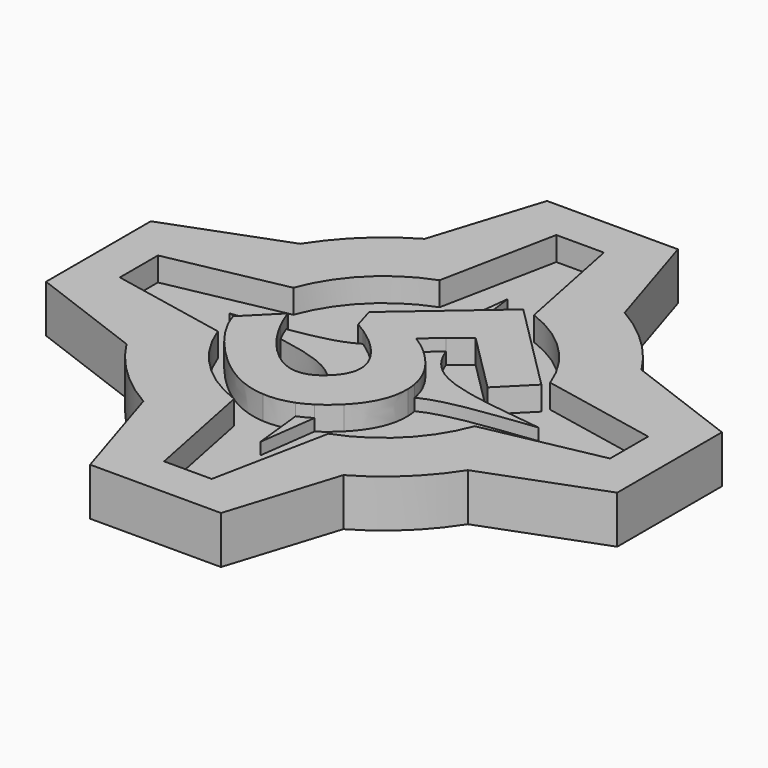
from build123d import *

# Parameters (mm, degrees)
F1_DEPTH = 2
F2_DEPTH = 1
F3_DEPTH = 1.5


# Not quite as in the source:
# - a feature names something its author has since deleted; it is built from what else it names


with BuildPart() as f1:
    # F0 (on Top) → F1 (new body)
    with BuildSketch(Plane.XY):
        with BuildLine():
            Line((-2.75, 12), (-4.2021191449, 7.3886531041))
            ThreePointArc((-4.2021191449, 7.3886531041), (-5.8600472341, 6.1570972393), (-7.1720131073, 4.5620420853))
            Line((-7.1720131073, 4.5620420853), (-12, 2.75))
            Line((-12, 2.75), (-12, -2.75))
            Line((-12, -2.75), (-7.1720131073, -4.5620420853))
            ThreePointArc((-7.1720131073, -4.5620420853), (-5.8600472341, -6.1570972393), (-4.2021191449, -7.3886531041))
            Line((-4.2021191449, -7.3886531041), (-2.75, -12))
            Line((-2.75, -12), (2.75, -12))
            Line((2.75, -12), (4.2021191449, -7.3886531041))
            ThreePointArc((4.2021191449, -7.3886531041), (5.8600472341, -6.1570972393), (7.1720131073, -4.5620420853))
            Line((7.1720131073, -4.5620420853), (12, -2.75))
            Line((12, -2.75), (12, 2.75))
            Line((12, 2.75), (7.1720131073, 4.5620420853))
            ThreePointArc((7.1720131073, 4.5620420853), (5.8600472341, 6.1570972393), (4.2021191449, 7.3886531041))
            Line((4.2021191449, 7.3886531041), (2.75, 12))
            Line((2.75, 12), (-2.75, 12))
        make_face()
        with BuildLine():
            ThreePointArc((-5.3974610581, 1.9824011012), (-4.0658639918, 4.0658639918), (-1.9824011012, 5.3974610581))
            Line((-1.9824011012, 5.3974610581), (-1, 10.3))
            Line((-1, 10.3), (1, 10.3))
            Line((1, 10.3), (1.9824011012, 5.3974610581))
            ThreePointArc((1.9824011012, 5.3974610581), (4.0658639918, 4.0658639918), (5.3974610581, 1.9824011012))
            Line((5.3974610581, 1.9824011012), (10.3, 1))
            Line((10.3, 1), (10.3, -1))
            Line((10.3, -1), (5.3974610581, -1.9824011012))
            ThreePointArc((5.3974610581, -1.9824011012), (4.0658639918, -4.0658639918), (1.9824011012, -5.3974610581))
            Line((1.9824011012, -5.3974610581), (1, -10.3))
            Line((1, -10.3), (-1, -10.3))
            Line((-1, -10.3), (-1.9824011012, -5.3974610581))
            ThreePointArc((-1.9824011012, -5.3974610581), (-4.0658639918, -4.0658639918), (-5.3974610581, -1.9824011012))
            Line((-5.3974610581, -1.9824011012), (-10.3, -1))
            Line((-10.3, -1), (-10.3, 1))
            Line((-10.3, 1), (-5.3974610581, 1.9824011012))
        make_face(mode=Mode.SUBTRACT)
    extrude(amount=F1_DEPTH)


with BuildPart() as f1b:
    # F0 (on Top) → F1, piece 2 (new body)
    with BuildSketch(Plane.XY):
        with BuildLine():
            Line((1.4579168065, 5.4941121132), (0.2654571044, 4.46607152))
            add(Edge.make_bspline(
                [(0.7478959675, 2.3141081763), (0.5408536455, 2.8552696341), (0.3998514188, 3.5527800211), (0.2654571044, 4.46607152)],
                knots=[6.0401561985, 6.0401561985, 6.0401561985, 6.0401561985, 7.9623527609, 7.9623527609, 7.9623527609, 7.9623527609], degree=3))
            Line((0.7478959675, 2.3141081763), (1.5004693947, 2.9375949951))
            Line((1.5004693947, 2.9375949951), (4.0028660863, 0.4343877588))
            Line((4.0028660863, 0.4343877588), (5.2598413938, 1.6909560547))
            Line((5.2598413938, 1.6909560547), (1.4579168065, 5.4941121132))
        make_face()
        with BuildLine():
            add(Edge.make_bspline(
                [(-0.7099336682, -2.2396454304), (-0.6256818584, -2.1704916087), (-0.5427903728, -2.0876269636)],
                knots=[0.925504666, 0.925504666, 0.925504666, 1, 1, 1], degree=2))
            add(Edge.make_bspline(
                [(-0.7099336682, -2.2396454304), (-0.4881454517, -2.7630250257), (-0.3518820462, -3.4434694111), (-0.2338863041, -4.3482357339)],
                knots=[5.8413396547, 5.8413396547, 5.8413396547, 5.8413396547, 7.8444431249, 7.8444431249, 7.8444431249, 7.8444431249], degree=3))
            add(Edge.make_bspline(
                [(0.3290608575, -4.0601655454), (0.0522382207, -4.2361734258), (-0.2338863041, -4.3482357339)],
                knots=[0.309252581, 0.309252581, 0.309252581, 0.5341322792, 0.5341322792, 0.5341322792], degree=2))
            add(Edge.make_bspline(
                [(0.3290608575, -4.0601655454), (0.6228480721, -2.2554562931), (0.987071243, -1.3852263771), (1.9925938258, -0.8786123417)],
                knots=[1.5244578408, 1.5244578408, 1.5244578408, 1.5244578408, 5.6104856332, 5.6104856332, 5.6104856332, 5.6104856332], degree=3))
            add(Edge.make_bspline(
                [(0.987609764, 0.8998355547), (1.8233684173, 0.0638061932), (1.9925938258, -0.8786123417)],
                knots=[0, 0, 0, 0.8228500432, 0.8228500432, 0.8228500432], degree=2))
            add(Edge.make_bspline(
                [(0.1959038432, 1.5567382899), (0.556479494, 1.331105471), (0.987609764, 0.8998355547)],
                knots=[0, 0, 0, 1, 1, 1], degree=2))
            Line((0.1959038432, 1.5567382899), (-0.0050966464, 1.6902740726))
            Line((-0.0050966464, 1.6902740726), (0.7478959675, 2.3141081763))
            add(Edge.make_bspline(
                [(0.7478959675, 2.3141081763), (0.5408536455, 2.8552696341), (0.3998514188, 3.5527800211), (0.2654571044, 4.46607152)],
                knots=[6.0401561985, 6.0401561985, 6.0401561985, 6.0401561985, 7.9623527609, 7.9623527609, 7.9623527609, 7.9623527609], degree=3))
            Line((0.2654571044, 4.46607152), (-0.3272992398, 3.9550457951))
            add(Edge.make_bspline(
                [(-0.3272992398, 3.9550457951), (-0.5803192593, 2.3906018232), (-0.9091205356, 1.5574827335), (-1.7244009065, 1.0449906882)],
                knots=[1.621694993, 1.621694993, 1.621694993, 1.621694993, 5.2829617669, 5.2829617669, 5.2829617669, 5.2829617669], degree=3))
            add(Edge.make_bspline(
                [(-1.4983144688, 0.8879619345), (-1.6173066461, 0.9732773429), (-1.7244009065, 1.0449906882)],
                knots=[0, 0, 0, 0.3328437229, 0.3328437229, 0.3328437229], degree=2))
            add(Edge.make_bspline(
                [(-0.8876580426, 0.3784024309), (-1.1408128274, 0.6316392144), (-1.4983144688, 0.8879619345)],
                knots=[0, 0, 0, 1, 1, 1], degree=2))
            add(Edge.make_bspline(
                [(-0.5427903728, -2.0876269636), (0.5177345813, -1.02744541), (-0.8876580426, 0.3784024309)],
                knots=[0, 0, 0, 1, 1, 1], degree=2))
        make_face()
        with BuildLine():
            add(Edge.make_bspline(
                [(-1.7244009065, 1.0449906882), (-1.9390620317, 1.1887338482), (-2.1059212368, 1.2778283886)],
                knots=[0.3328437229, 0.3328437229, 0.3328437229, 1, 1, 1], degree=2))
            add(Edge.make_bspline(
                [(-0.3272992398, 3.9550457951), (-0.5803192593, 2.3906018232), (-0.9091205356, 1.5574827335), (-1.7244009065, 1.0449906882)],
                knots=[1.621694993, 1.621694993, 1.621694993, 1.621694993, 5.2829617669, 5.2829617669, 5.2829617669, 5.2829617669], degree=3))
            Line((-0.3272992398, 3.9550457951), (-2.3789186791, 2.1863084016))
            Line((-2.3789186791, 2.1863084016), (-2.1059212368, 1.2778283886))
        make_face()
        with BuildLine():
            add(Edge.make_bspline(
                [(0.3290608575, -4.0601655454), (0.6228480721, -2.2554562931), (0.987071243, -1.3852263771), (1.9925938258, -0.8786123417)],
                knots=[1.5244578408, 1.5244578408, 1.5244578408, 1.5244578408, 5.6104856332, 5.6104856332, 5.6104856332, 5.6104856332], degree=3))
            add(Edge.make_bspline(
                [(1.07283769, -3.4551458487), (0.7097449104, -3.818121058), (0.3290608575, -4.0601655454)],
                knots=[0, 0, 0, 0.309252581, 0.309252581, 0.309252581], degree=2))
            add(Edge.make_bspline(
                [(2.0345651408, -1.289326677), (2.0658328352, -2.4624722377), (1.07283769, -3.4551458487)],
                knots=[0, 0, 0, 1, 1, 1], degree=2))
            add(Edge.make_bspline(
                [(1.9925938258, -0.8786123417), (2.0290260701, -1.0815039915), (2.0345651408, -1.289326677)],
                knots=[0.8228500432, 0.8228500432, 0.8228500432, 1, 1, 1], degree=2))
        make_face()
        with BuildLine():
            add(Edge.make_bspline(
                [(-5.0476920503, -0.2054319436), (-4.6911689085, -0.2581182841), (-4.3627018531, -0.3095354756), (-4.0598230569, -0.3621513456)],
                knots=[0.8212011644, 0.8212011644, 0.8212011644, 0.8212011644, 1.4868249386, 1.4868249386, 1.4868249386, 1.4868249386], degree=3))
            Line((-5.0476920503, -0.2054319436), (-5.6740216756, -0.8315587618))
            add(Edge.make_bspline(
                [(-4.1644213444, -3.0998236856), (-5.3350704405, -1.9287954077), (-5.6740216756, -0.8315587618)],
                knots=[0, 0, 0, 1, 1, 1], degree=2))
            add(Edge.make_bspline(
                [(-1.4592955796, -4.5381069077), (-2.8173310346, -4.4473503278), (-4.1644213444, -3.0998236856)],
                knots=[0, 0, 0, 1, 1, 1], degree=2))
            add(Edge.make_bspline(
                [(-0.2338863041, -4.3482357339), (-0.8266306975, -4.5803874688), (-1.4592955796, -4.5381069077)],
                knots=[0.5341322792, 0.5341322792, 0.5341322792, 1, 1, 1], degree=2))
            add(Edge.make_bspline(
                [(-0.7099336682, -2.2396454304), (-0.4881454517, -2.7630250257), (-0.3518820462, -3.4434694111), (-0.2338863041, -4.3482357339)],
                knots=[5.8413396547, 5.8413396547, 5.8413396547, 5.8413396547, 7.8444431249, 7.8444431249, 7.8444431249, 7.8444431249], degree=3))
            add(Edge.make_bspline(
                [(-3.0133276619, -1.8417037247), (-1.7566494671, -3.0987889667), (-0.7099336682, -2.2396454304)],
                knots=[0, 0, 0, 0.925504666, 0.925504666, 0.925504666], degree=2))
            add(Edge.make_bspline(
                [(-3.8394915756, -0.7605006452), (-3.4628691889, -1.3920165878), (-3.0133276619, -1.8417037247)],
                knots=[0, 0, 0, 1, 1, 1], degree=2))
            add(Edge.make_bspline(
                [(-4.0598230569, -0.3621513456), (-3.9598892689, -0.5586192237), (-3.8394915756, -0.7605006452)],
                knots=[0.6803225258, 0.6803225258, 0.6803225258, 1, 1, 1], degree=2))
        make_face()
        with BuildLine():
            Line((-4.5875235257, 0.2545875773), (-5.0476920503, -0.2054319436))
            add(Edge.make_bspline(
                [(-5.0476920503, -0.2054319436), (-4.6911689085, -0.2581182841), (-4.3627018531, -0.3095354756), (-4.0598230569, -0.3621513456)],
                knots=[0.8212011644, 0.8212011644, 0.8212011644, 0.8212011644, 1.4868249386, 1.4868249386, 1.4868249386, 1.4868249386], degree=3))
            add(Edge.make_bspline(
                [(-4.3409756358, 0.2916852868), (-4.2301083517, -0.0273737774), (-4.0598230569, -0.3621513456)],
                knots=[0.1355981238, 0.1355981238, 0.1355981238, 0.6803225258, 0.6803225258, 0.6803225258], degree=2))
            add(Edge.make_bspline(
                [(-4.3409756358, 0.2916852868), (-4.4214269269, 0.2792690242), (-4.5035953579, 0.26691732), (-4.5875235257, 0.2545875773)],
                knots=[7.8805599952, 7.8805599952, 7.8805599952, 7.8805599952, 8.0525816561, 8.0525816561, 8.0525816561, 8.0525816561], degree=3))
        make_face()
        with BuildLine():
            Line((-4.3924900739, 0.4495578768), (-4.5875235257, 0.2545875773))
            add(Edge.make_bspline(
                [(-4.3409756358, 0.2916852868), (-4.4214269269, 0.2792690242), (-4.5035953579, 0.26691732), (-4.5875235257, 0.2545875773)],
                knots=[7.8805599952, 7.8805599952, 7.8805599952, 7.8805599952, 8.0525816561, 8.0525816561, 8.0525816561, 8.0525816561], degree=3))
            add(Edge.make_bspline(
                [(-4.3924900739, 0.4495578768), (-4.3685738041, 0.3711085885), (-4.3409756358, 0.2916852868)],
                knots=[0, 0, 0, 0.1355981238, 0.1355981238, 0.1355981238], degree=2))
        make_face()
    extrude(amount=F1_DEPTH)


with BuildPart() as f2:
    # F0 (on Top) → F2 (new body)
    with BuildSketch(Plane.XY):
        with BuildLine():
            Line((-1, 10.3), (-1.9824011012, 5.3974610581))
            ThreePointArc((-1.9824011012, 5.3974610581), (-4.0658639918, 4.0658639918), (-5.3974610581, 1.9824011012))
            Line((-5.3974610581, 1.9824011012), (-10.3, 1))
            Line((-10.3, 1), (-10.3, -1))
            Line((-10.3, -1), (-5.3974610581, -1.9824011012))
            ThreePointArc((-5.3974610581, -1.9824011012), (-4.0658639918, -4.0658639918), (-1.9824011012, -5.3974610581))
            Line((-1.9824011012, -5.3974610581), (-1, -10.3))
            Line((-1, -10.3), (1, -10.3))
            Line((1, -10.3), (1.9824011012, -5.3974610581))
            ThreePointArc((1.9824011012, -5.3974610581), (4.0658639918, -4.0658639918), (5.3974610581, -1.9824011012))
            Line((5.3974610581, -1.9824011012), (10.3, -1))
            Line((10.3, -1), (10.3, 1))
            Line((10.3, 1), (5.3974610581, 1.9824011012))
            ThreePointArc((5.3974610581, 1.9824011012), (4.0658639918, 4.0658639918), (1.9824011012, 5.3974610581))
            Line((1.9824011012, 5.3974610581), (1, 10.3))
            Line((1, 10.3), (-1, 10.3))
        make_face()
        with BuildLine():
            add(Edge.make_bspline(
                [(-6.5, 0), (-5.9701038682, -0.0734985607), (-5.4875459594, -0.1404311341), (-5.0476920503, -0.2054319436)],
                knots=[0, 0, 0, 0, 0.8212011644, 0.8212011644, 0.8212011644, 0.8212011644], degree=3))
            add(Edge.make_bspline(
                [(-4.5875235257, 0.2545875773), (-5.1436271619, 0.1728913493), (-5.7769888409, 0.0921593026), (-6.5, 0)],
                knots=[8.0525816561, 8.0525816561, 8.0525816561, 8.0525816561, 9.1923881554, 9.1923881554, 9.1923881554, 9.1923881554], degree=3))
            Line((-4.5875235257, 0.2545875773), (-4.3924900739, 0.4495578768))
            add(Edge.make_bspline(
                [(-4.3924900739, 0.4495578768), (-4.3685738041, 0.3711085885), (-4.3409756358, 0.2916852868)],
                knots=[0, 0, 0, 0.1355981238, 0.1355981238, 0.1355981238], degree=2))
            add(Edge.make_bspline(
                [(-1.7244009065, 1.0449906882), (-2.3028266202, 0.6813874572), (-3.1261278658, 0.4791759876), (-4.3409756358, 0.2916852868)],
                knots=[5.2829617669, 5.2829617669, 5.2829617669, 5.2829617669, 7.8805599952, 7.8805599952, 7.8805599952, 7.8805599952], degree=3))
            add(Edge.make_bspline(
                [(-1.7244009065, 1.0449906882), (-1.9390620317, 1.1887338482), (-2.1059212368, 1.2778283886)],
                knots=[0.3328437229, 0.3328437229, 0.3328437229, 1, 1, 1], degree=2))
            Line((-2.1059212368, 1.2778283886), (-2.3789186791, 2.1863084016))
            Line((-2.3789186791, 2.1863084016), (-0.3272992398, 3.9550457951))
            add(Edge.make_bspline(
                [(0, 6.5), (-0.1180250107, 5.4844109751), (-0.2152283845, 4.6479892796), (-0.3272992398, 3.9550457951)],
                knots=[0, 0, 0, 0, 1.621694993, 1.621694993, 1.621694993, 1.621694993], degree=3))
            add(Edge.make_bspline(
                [(0.2654571044, 4.46607152), (0.1794566574, 5.0504971147), (0.0961620616, 5.7232821691), (0, 6.5)],
                knots=[7.9623527609, 7.9623527609, 7.9623527609, 7.9623527609, 9.1923881554, 9.1923881554, 9.1923881554, 9.1923881554], degree=3))
            Line((0.2654571044, 4.46607152), (1.4579168065, 5.4941121132))
            Line((1.4579168065, 5.4941121132), (5.2598413938, 1.6909560547))
            Line((5.2598413938, 1.6909560547), (4.0028660863, 0.4343877588))
            Line((4.0028660863, 0.4343877588), (1.5004693947, 2.9375949951))
            Line((1.5004693947, 2.9375949951), (0.7478959675, 2.3141081763))
            add(Edge.make_bspline(
                [(6.5, 0), (2.7011736647, 0.4569199424), (1.3984891424, 0.6136058459), (0.7478959675, 2.3141081763)],
                knots=[0, 0, 0, 0, 6.0401561985, 6.0401561985, 6.0401561985, 6.0401561985], degree=3))
            add(Edge.make_bspline(
                [(1.9925938258, -0.8786123417), (2.8740572073, -0.4345032502), (4.2483376502, -0.2698207515), (6.5, 0)],
                knots=[5.6104856332, 5.6104856332, 5.6104856332, 5.6104856332, 9.1923881554, 9.1923881554, 9.1923881554, 9.1923881554], degree=3))
            add(Edge.make_bspline(
                [(1.9925938258, -0.8786123417), (2.0290260701, -1.0815039915), (2.0345651408, -1.289326677)],
                knots=[0.8228500432, 0.8228500432, 0.8228500432, 1, 1, 1], degree=2))
            add(Edge.make_bspline(
                [(2.0345651408, -1.289326677), (2.0658328352, -2.4624722377), (1.07283769, -3.4551458487)],
                knots=[0, 0, 0, 1, 1, 1], degree=2))
            add(Edge.make_bspline(
                [(1.07283769, -3.4551458487), (0.7097449104, -3.818121058), (0.3290608575, -4.0601655454)],
                knots=[0, 0, 0, 0.309252581, 0.309252581, 0.309252581], degree=2))
            add(Edge.make_bspline(
                [(0, -6.5), (0.1196469007, -5.5368812446), (0.2194516611, -4.7334852852), (0.3290608575, -4.0601655454)],
                knots=[0, 0, 0, 0, 1.5244578408, 1.5244578408, 1.5244578408, 1.5244578408], degree=3))
            add(Edge.make_bspline(
                [(-0.2338863041, -4.3482357339), (-0.154483629, -4.9570786054), (-0.0833531458, -5.6675017426), (0, -6.5)],
                knots=[7.8444431249, 7.8444431249, 7.8444431249, 7.8444431249, 9.1923881554, 9.1923881554, 9.1923881554, 9.1923881554], degree=3))
            add(Edge.make_bspline(
                [(-0.2338863041, -4.3482357339), (-0.8266306975, -4.5803874688), (-1.4592955796, -4.5381069077)],
                knots=[0.5341322792, 0.5341322792, 0.5341322792, 1, 1, 1], degree=2))
            add(Edge.make_bspline(
                [(-1.4592955796, -4.5381069077), (-2.8173310346, -4.4473503278), (-4.1644213444, -3.0998236856)],
                knots=[0, 0, 0, 1, 1, 1], degree=2))
            add(Edge.make_bspline(
                [(-4.1644213444, -3.0998236856), (-5.3350704405, -1.9287954077), (-5.6740216756, -0.8315587618)],
                knots=[0, 0, 0, 1, 1, 1], degree=2))
            Line((-5.6740216756, -0.8315587618), (-5.0476920503, -0.2054319436))
        make_face(mode=Mode.SUBTRACT)
    extrude(amount=F2_DEPTH)


with BuildPart() as f3:
    # F0 (on Top) → F3 (new body)
    with BuildSketch(Plane.XY):
        with BuildLine():
            add(Edge.make_bspline(
                [(0, 6.5), (-0.1180250107, 5.4844109751), (-0.2152283845, 4.6479892796), (-0.3272992398, 3.9550457951)],
                knots=[0, 0, 0, 0, 1.621694993, 1.621694993, 1.621694993, 1.621694993], degree=3))
            Line((-0.3272992398, 3.9550457951), (0.2654571044, 4.46607152))
            add(Edge.make_bspline(
                [(0.2654571044, 4.46607152), (0.1794566574, 5.0504971147), (0.0961620616, 5.7232821691), (0, 6.5)],
                knots=[7.9623527609, 7.9623527609, 7.9623527609, 7.9623527609, 9.1923881554, 9.1923881554, 9.1923881554, 9.1923881554], degree=3))
        make_face()
    extrude(amount=F3_DEPTH)


with BuildPart() as f3b:
    # F0 (on Top) → F3, piece 2 (new body)
    with BuildSketch(Plane.XY):
        with BuildLine():
            add(Edge.make_bspline(
                [(0.987609764, 0.8998355547), (1.8233684173, 0.0638061932), (1.9925938258, -0.8786123417)],
                knots=[0, 0, 0, 0.8228500432, 0.8228500432, 0.8228500432], degree=2))
            add(Edge.make_bspline(
                [(1.9925938258, -0.8786123417), (2.8740572073, -0.4345032502), (4.2483376502, -0.2698207515), (6.5, 0)],
                knots=[5.6104856332, 5.6104856332, 5.6104856332, 5.6104856332, 9.1923881554, 9.1923881554, 9.1923881554, 9.1923881554], degree=3))
            add(Edge.make_bspline(
                [(6.5, 0), (2.7011736647, 0.4569199424), (1.3984891424, 0.6136058459), (0.7478959675, 2.3141081763)],
                knots=[0, 0, 0, 0, 6.0401561985, 6.0401561985, 6.0401561985, 6.0401561985], degree=3))
            Line((0.7478959675, 2.3141081763), (-0.0050966464, 1.6902740726))
            Line((-0.0050966464, 1.6902740726), (0.1959038432, 1.5567382899))
            add(Edge.make_bspline(
                [(0.1959038432, 1.5567382899), (0.556479494, 1.331105471), (0.987609764, 0.8998355547)],
                knots=[0, 0, 0, 1, 1, 1], degree=2))
        make_face()
    extrude(amount=F3_DEPTH)


with BuildPart() as f3c:
    # F0 (on Top) → F3, piece 3 (new body)
    with BuildSketch(Plane.XY):
        with BuildLine():
            add(Edge.make_bspline(
                [(-4.3409756358, 0.2916852868), (-4.2301083517, -0.0273737774), (-4.0598230569, -0.3621513456)],
                knots=[0.1355981238, 0.1355981238, 0.1355981238, 0.6803225258, 0.6803225258, 0.6803225258], degree=2))
            add(Edge.make_bspline(
                [(-4.0598230569, -0.3621513456), (-2.0783881585, -0.706364682), (-1.1920755379, -1.1018788679), (-0.7099336682, -2.2396454304)],
                knots=[1.4868249386, 1.4868249386, 1.4868249386, 1.4868249386, 5.8413396547, 5.8413396547, 5.8413396547, 5.8413396547], degree=3))
            add(Edge.make_bspline(
                [(-0.7099336682, -2.2396454304), (-0.6256818584, -2.1704916087), (-0.5427903728, -2.0876269636)],
                knots=[0.925504666, 0.925504666, 0.925504666, 1, 1, 1], degree=2))
            add(Edge.make_bspline(
                [(-0.5427903728, -2.0876269636), (0.5177345813, -1.02744541), (-0.8876580426, 0.3784024309)],
                knots=[0, 0, 0, 1, 1, 1], degree=2))
            add(Edge.make_bspline(
                [(-0.8876580426, 0.3784024309), (-1.1408128274, 0.6316392144), (-1.4983144688, 0.8879619345)],
                knots=[0, 0, 0, 1, 1, 1], degree=2))
            add(Edge.make_bspline(
                [(-1.4983144688, 0.8879619345), (-1.6173066461, 0.9732773429), (-1.7244009065, 1.0449906882)],
                knots=[0, 0, 0, 0.3328437229, 0.3328437229, 0.3328437229], degree=2))
            add(Edge.make_bspline(
                [(-1.7244009065, 1.0449906882), (-2.3028266202, 0.6813874572), (-3.1261278658, 0.4791759876), (-4.3409756358, 0.2916852868)],
                knots=[5.2829617669, 5.2829617669, 5.2829617669, 5.2829617669, 7.8805599952, 7.8805599952, 7.8805599952, 7.8805599952], degree=3))
        make_face()
    extrude(amount=F3_DEPTH)


with BuildPart() as f3d:
    # F0 (on Top) → F3, piece 4 (new body)
    with BuildSketch(Plane.XY):
        with BuildLine():
            add(Edge.make_bspline(
                [(0.3290608575, -4.0601655454), (0.0522382207, -4.2361734258), (-0.2338863041, -4.3482357339)],
                knots=[0.309252581, 0.309252581, 0.309252581, 0.5341322792, 0.5341322792, 0.5341322792], degree=2))
            add(Edge.make_bspline(
                [(-0.2338863041, -4.3482357339), (-0.154483629, -4.9570786054), (-0.0833531458, -5.6675017426), (0, -6.5)],
                knots=[7.8444431249, 7.8444431249, 7.8444431249, 7.8444431249, 9.1923881554, 9.1923881554, 9.1923881554, 9.1923881554], degree=3))
            add(Edge.make_bspline(
                [(0, -6.5), (0.1196469007, -5.5368812446), (0.2194516611, -4.7334852852), (0.3290608575, -4.0601655454)],
                knots=[0, 0, 0, 0, 1.5244578408, 1.5244578408, 1.5244578408, 1.5244578408], degree=3))
        make_face()
    extrude(amount=F3_DEPTH)


with BuildPart() as f3e:
    # F0 (on Top) → F3, piece 5 (new body)
    with BuildSketch(Plane.XY):
        with BuildLine():
            add(Edge.make_bspline(
                [(-4.5875235257, 0.2545875773), (-5.1436271619, 0.1728913493), (-5.7769888409, 0.0921593026), (-6.5, 0)],
                knots=[8.0525816561, 8.0525816561, 8.0525816561, 8.0525816561, 9.1923881554, 9.1923881554, 9.1923881554, 9.1923881554], degree=3))
            add(Edge.make_bspline(
                [(-6.5, 0), (-5.9701038682, -0.0734985607), (-5.4875459594, -0.1404311341), (-5.0476920503, -0.2054319436)],
                knots=[0, 0, 0, 0, 0.8212011644, 0.8212011644, 0.8212011644, 0.8212011644], degree=3))
            Line((-5.0476920503, -0.2054319436), (-4.5875235257, 0.2545875773))
        make_face()
    extrude(amount=F3_DEPTH)


solid = Compound([f1.part, f1b.part, f2.part, f3.part, f3b.part, f3c.part, f3d.part, f3e.part])
